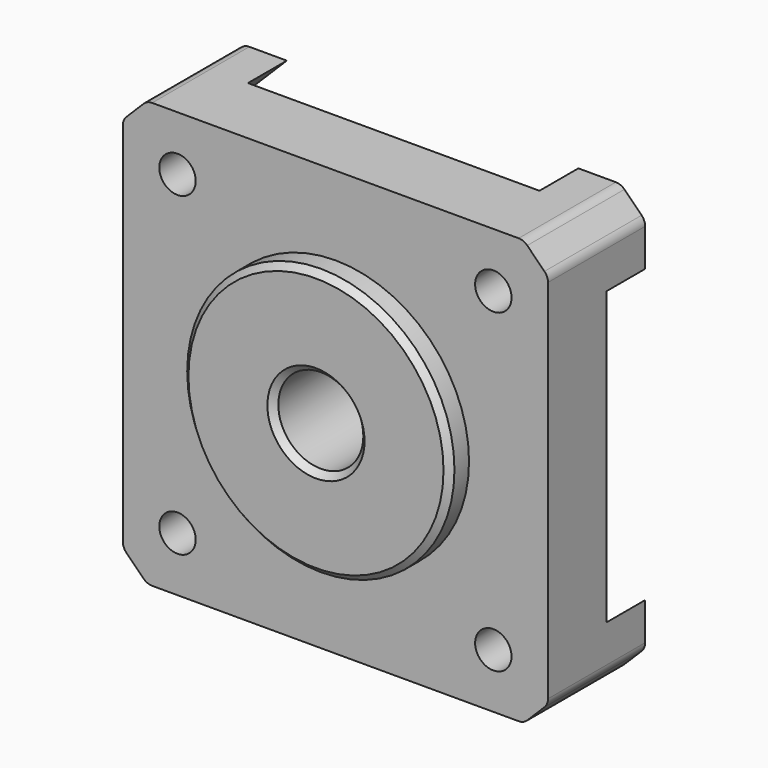
from build123d import *

# Parameters (mm, degrees)
F0_W      = 35
F0_H      = 35
F1_DEPTH  = 10
F2_SIZE   = 2
F3_R      = 11
F4_DEPTH  = 0.5
F5_R      = 11
F6_DEPTH  = 2.5
F7_R      = 3.5
F8_DEPTH  = 12.001
F9_R      = 1
F10_SIZE  = 0.5
F11_R     = 1.5
F12_DEPTH = 10.001
F14_DEPTH = 4


with BuildPart() as f1:
    # F0 (on Front) → F1 (new body)
    with BuildSketch(Plane.XZ):
        Rectangle(F0_W, F0_H)
    extrude(amount=F1_DEPTH)

    # F2
    f2_edges = [f1.edges().sort_by_distance(p)[0] for p in [
        (-17.5, -5, 17.5),
        (17.5, -5, 17.5),
        (17.5, -5, -17.5),
        (-17.5, -5, -17.5),
    ]]
    chamfer(f2_edges, length=F2_SIZE)

    # F3 (on face) → F4 (cut)
    with BuildSketch(Plane.XZ.offset(10)):
        Circle(F3_R)
    extrude(amount=-F4_DEPTH, mode=Mode.SUBTRACT)

    # F5 (on face) → F6 (join)
    with BuildSketch(Plane.XZ.offset(9.5)):
        Circle(F5_R)
    extrude(amount=F6_DEPTH)

    # F7 (on face) → F8 (cut, through all)
    with BuildSketch(Plane.XZ.offset(12)):
        Circle(F7_R)
    extrude(amount=-F8_DEPTH, mode=Mode.SUBTRACT)

    # F9
    f9_edges = [f1.edges().sort_by_distance(p)[0] for p in [
        (-15.5, -5, 17.5),
        (15.5, -5, 17.5),
        (17.5, -5, 15.5),
        (17.5, -5, -15.5),
        (15.5, -5, -17.5),
        (-15.5, -5, -17.5),
        (-17.5, -5, -15.5),
        (-17.5, -5, 15.5),
    ]]
    fillet(f9_edges, radius=F9_R)

    # F10
    f10_edges = [f1.edges().sort_by_distance(p)[0] for p in [
        (-11, -12, 0),
        (-3.5, -12, 0),
    ]]
    chamfer(f10_edges, length=F10_SIZE)

    # F11 (on face) → F12 (cut, through all)
    with BuildSketch(Plane.XZ.offset(10)):
        with Locations((-13, 13)):
            Circle(F11_R)
        with Locations((-13, -13)):
            Circle(F11_R)
        with Locations((13, -13)):
            Circle(F11_R)
        with Locations((13, 13)):
            Circle(F11_R)
    extrude(amount=-F12_DEPTH, mode=Mode.SUBTRACT)

    # F13 (on face) → F14 (cut)
    with BuildSketch(Plane(origin=(0, 0, 0), x_dir=(-1, 0, 0), z_dir=(0, 1, 0))):
        Polygon((12, 17.5), (-12, 17.5), (-17.5, 12), (-17.5, -12), (-12, -17.5), (12, -17.5), (17.5, -12), (17.5, 12), align=None)
    extrude(amount=-F14_DEPTH, mode=Mode.SUBTRACT)


solid = f1.part
